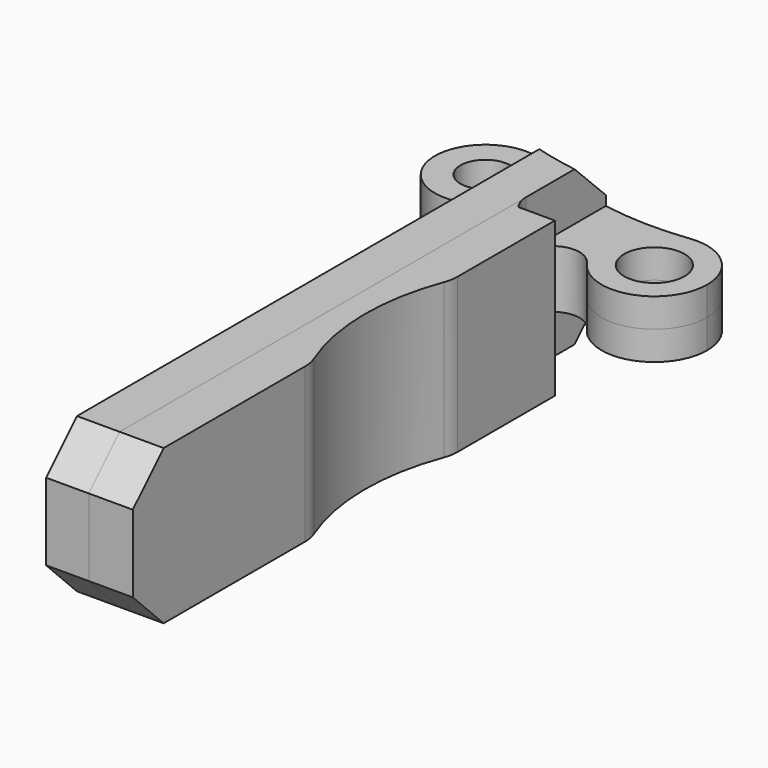
from build123d import *

# Parameters (mm, degrees)
F0_W        = 5.6202424753
F0_H        = 7.3923990308
F1_DEPTH    = 10.16
F0_R        = 3.2880029728
F0_R_2      = 3.9763748147
F2_DEPTH    = 3.81
F3_SIZE     = 5.08
F4_DEPTH    = 10.16
F5_SIZE     = 5.08
F6_T1_DEPTH = 7.62
F6_2_F1_R   = 5.08
F6_2_F2_R   = 5.08
F8_DEPTH    = 12.7


# Not quite as in the source:
# - a fillet or chamfer that OpenCascade refuses, or shapes differently, is made with other operations: its cross-section is extruded or revolved along the edge and cut away or added


with BuildPart() as f1:
    # F0 (on Top) → F1 (new body, symmetric)
    with BuildSketch(Plane.XY):
        Polygon((-23.8571265649, 38.1211079657), (-29.4773678438, 38.1211079657), (-29.4773678438, 33.8620854561), (-29.4773689242, -34.9397621871), (-23.8571265649, -34.9397622754), (-23.8571265649, 29.6442432214), align=None)
        with BuildLine():
            ThreePointArc((-23.8571265649, 42.7830699379), (-26.6935732854, 43.3808072311), (-29.4773678438, 44.1890199055))
            Line((-29.4773678438, 44.1890199055), (-29.4773678438, 38.1211079657))
            Line((-29.4773678438, 38.1211079657), (-23.8571265649, 38.1211079657))
            Line((-23.8571265649, 38.1211079657), (-23.8571265649, 42.7830699379))
        make_face()
        with Locations((-26.6672478026, -38.6359617025)):
            Rectangle(F0_W, F0_H)
    extrude(amount=F1_DEPTH, both=True)

    # F0 (on Top) → F2 (join, symmetric)
    with BuildSketch(Plane.XY):
        with BuildLine():
            ThreePointArc((-31.6869179481, 38.1211079657), (-31.3536995737, 39.297400699), (-31.2413621678, 40.5148075278))
            ThreePointArc((-31.2413621678, 40.5148075278), (-32.2218622797, 43.9910999495), (-34.8743439371, 46.4426974955))
            ThreePointArc((-34.8743439371, 46.4426974955), (-44.1066653776, 38.1351969368), (-31.6869179481, 38.1211079657))
        make_face()
        with Locations((-37.8940842395, 40.5148075278)):
            Circle(F0_R, mode=Mode.SUBTRACT)
        with BuildLine():
            ThreePointArc((-4.763312552, 35.6086244195), (-7.1105593997, 40.8187113422), (-12.5681646531, 42.5125585623))
            ThreePointArc((-12.5681646531, 42.5125585623), (-18.0664915689, 38.4542200705), (-17.4383845866, 31.6492812901))
            ThreePointArc((-17.4383845866, 31.6492812901), (-9.6452347995, 28.9690866137), (-4.763312552, 35.6086244195))
        make_face()
        with Locations((-11.7192433987, 35.6086244195)):
            Circle(F0_R_2, mode=Mode.SUBTRACT)
        with BuildLine():
            ThreePointArc((-12.5681646531, 42.5125585623), (-18.2225576344, 42.2341662967), (-23.8571265649, 42.7830699379))
            Line((-23.8571265649, 42.7830699379), (-23.8571265649, 38.1211079657))
            Line((-23.8571265649, 38.1211079657), (-23.8571265649, 29.6442432214))
            ThreePointArc((-23.8571265649, 29.6442432214), (-21.3848882076, 33.0065499535), (-17.4383845866, 31.6492812901))
            ThreePointArc((-17.4383845866, 31.6492812901), (-18.0664915689, 38.4542200705), (-12.5681646531, 42.5125585623))
        make_face()
        with BuildLine():
            ThreePointArc((-34.8743439371, 46.4426974955), (-32.2218622797, 43.9910999495), (-31.2413621678, 40.5148075278))
            ThreePointArc((-31.2413621678, 40.5148075278), (-31.3536995737, 39.297400699), (-31.6869179481, 38.1211079657))
            Line((-31.6869179481, 38.1211079657), (-29.4773678438, 38.1211079657))
            Line((-29.4773678438, 38.1211079657), (-29.4773678438, 44.1890199055))
            ThreePointArc((-29.4773678438, 44.1890199055), (-32.2184586739, 45.213836031), (-34.8743439371, 46.4426974955))
        make_face()
    extrude(amount=F2_DEPTH, both=True)

    # F3
    f3_edges = [f1.edges().sort_by_distance(p)[0] for p in [
        (-26.693573, 43.380807, 10.16),
        (-26.693573, 43.380807, -10.16),
        (-26.667248, -42.332161, 10.16),
        (-26.667248, -42.332161, -10.16),
    ]]
    chamfer(f3_edges, length=F3_SIZE)

    # F6: fillet of radius 5.08 on 4 edges, made by hand

    # F6_s2 → F6_t1 (join)
    with BuildSketch(Plane.XY.offset(-3.81)):
        with BuildLine():
            ThreePointArc((-29.4773678427, 33.9298172252), (-30.063578473, 36.2988375878), (-31.6869179481, 38.1211079657))
            Line((-31.6869179481, 38.1211079657), (-31.3998729586, 38.5402370318))
            ThreePointArc((-31.3998729586, 38.5402370318), (-30.5821428959, 38.6291079657), (-29.4773678438, 38.6291079657))
            Line((-29.4773678438, 38.6291079657), (-28.9693678438, 38.1211079657))
            Line((-28.9693678438, 38.1211079657), (-28.9693678427, 33.9298172173))
            Line((-28.9693678427, 33.9298172173), (-29.4773678427, 33.9298172252))
        make_face()
    extrude(amount=F6_T1_DEPTH)

    # F7 (on face) → F8 (cut)
    with BuildSketch(Plane(origin=(-29.4773683755, 4.629e-07, 0), x_dir=(-1.57e-08, -1, 0), z_dir=(-1, 1.57e-08, 0))):
        Polygon((36.3451056182, -7.62), (39.7921616808, -4.9903579056), (39.7921616808, 3.623371711), (36.7539399008, 7.5733514423), (28.3016198795, 7.443575354), (28.3016198795, -7.62), align=None)
        Polygon((9.9728746732, 7.1621576072), (22.8604692966, -7.62), (22.6305215634, 7.3565018696), align=None)
        Polygon((17.961487174, -7.62), (5.0967486238, 7.0872900485), (5.3225629052, -7.62), align=None)
        Polygon((0, -7.62), (0, 7.0090350727), (-14.8322781086, 6.7813017369), align=None)
        Polygon((-21.4508656455, 6.6796805964), (-20.3723220551, -7.62), (-8.6206179077, -7.62), align=None)
    extrude(amount=-F8_DEPTH, mode=Mode.SUBTRACT)


with BuildPart() as f4:
    # F0 (on Top) → F4 (new body, symmetric)
    with BuildSketch(Plane.XY):
        with BuildLine():
            ThreePointArc((-23.0891581237, 27.4486547619), (-23.6595960638, 28.481231591), (-23.8571265649, 29.6442432214))
            Line((-23.8571265649, 29.6442432214), (-23.8571265649, -34.9397622754))
            Line((-23.8571265649, -34.9397622754), (-23.8571265649, -42.3321612179))
            Line((-23.8571265649, -42.3321612179), (-18.0597770959, -42.3321612179))
            Line((-18.0597770959, -42.3321612179), (-18.0597770959, -12.9362130538))
            ThreePointArc((-18.0597770959, -12.9362130538), (-20.5510916383, -1.2707557569), (-18.2962100953, 10.442700237))
            Line((-18.2962100953, 10.442700237), (-18.2962100953, 27.4486547619))
            Line((-18.2962100953, 27.4486547619), (-23.0891581237, 27.4486547619))
        make_face()
    extrude(amount=F4_DEPTH, both=True)

    # F5
    f5_edges = [f4.edges().sort_by_distance(p)[0] for p in [
        (-20.958452, -42.332161, 10.16),
        (-20.958452, -42.332161, -10.16),
    ]]
    chamfer(f5_edges, length=F5_SIZE)

    # F6#2: fillet of radius 5.08 on 2 edges, made by hand

    # F6_2_f1
    f6_2_f1_edges = [f4.edges().sort_by_distance(p)[0] for p in [
        (-18.0597770959, -12.9362130538, 0),
    ]]
    fillet(f6_2_f1_edges, radius=F6_2_F1_R)

    # F6_2_f2
    f6_2_f2_edges = [f4.edges().sort_by_distance(p)[0] for p in [
        (-18.2962100953, 10.442700237, 0),
    ]]
    fillet(f6_2_f2_edges, radius=F6_2_F2_R)


solid = Compound([f1.part, f4.part])
